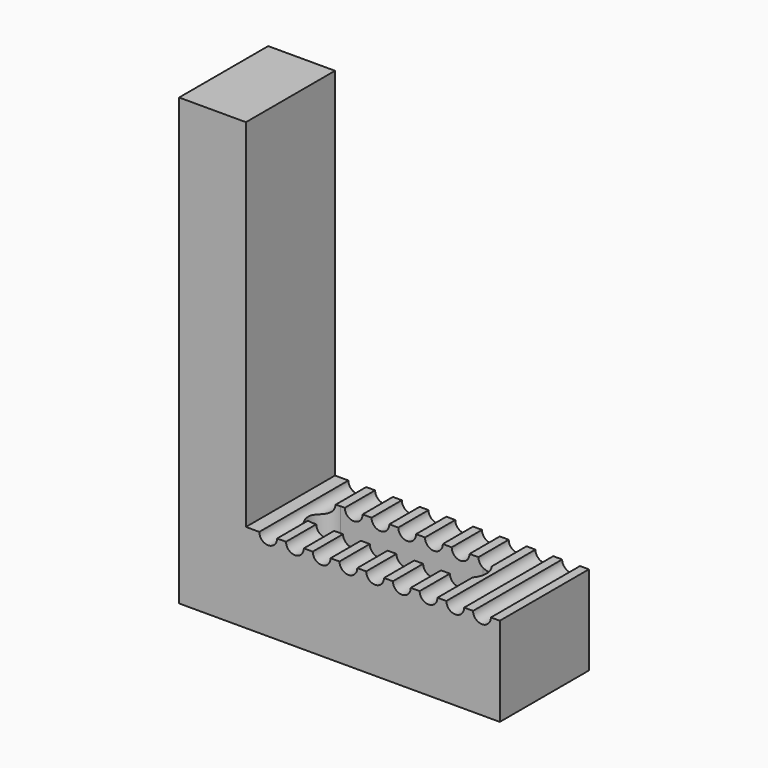
from build123d import *

# Parameters (mm, degrees)
F1_DEPTH = 15.875
F3_DEPTH = 25.4
F5_DEPTH = 25.4


with BuildPart() as f1:
    # F0 (on Front) → F1 (new body)
    with BuildSketch(Plane.XZ):
        Polygon((-45.72, 0), (0, 0), (0, 12.7), (-36.195, 12.7), (-36.195, 63.5), (-45.72, 63.5), align=None)
    extrude(amount=F1_DEPTH)

    # F2 (on face) → F3 (cut)
    with BuildSketch(Plane.XY.offset(12.7)):
        with BuildLine():
            Line((-10.795, -5.3975), (-31.115, -5.3975))
            ThreePointArc((-31.115, -5.3975), (-33.655, -7.9375), (-31.115, -10.4775))
            Line((-31.115, -10.4775), (-10.795, -10.4775))
            ThreePointArc((-10.795, -10.4775), (-8.255, -7.9375), (-10.795, -5.3975))
        make_face()
    extrude(amount=-F3_DEPTH, mode=Mode.SUBTRACT)

    # F4 (on face) → F5 (cut)
    with BuildSketch(Plane(origin=(0, 0, 0), x_dir=(-1, 0, 0), z_dir=(0, 1, 0))):
        with BuildLine():
            ThreePointArc((24.13, 12.7), (25.4, 11.43), (26.67, 12.7))
            Line((26.67, 12.7), (24.13, 12.7))
        make_face()
        with BuildLine():
            Line((30.48, 12.7), (27.94, 12.7))
            ThreePointArc((27.94, 12.7), (29.21, 11.43), (30.48, 12.7))
        make_face()
        with BuildLine():
            ThreePointArc((20.32, 12.7), (21.59, 11.43), (22.86, 12.7))
            Line((22.86, 12.7), (20.32, 12.7))
        make_face()
        with BuildLine():
            Line((34.29, 12.7), (31.75, 12.7))
            ThreePointArc((31.75, 12.7), (33.02, 11.43), (34.29, 12.7))
        make_face()
        with BuildLine():
            ThreePointArc((16.51, 12.7), (17.78, 11.43), (19.05, 12.7))
            Line((19.05, 12.7), (16.51, 12.7))
        make_face()
        with BuildLine():
            ThreePointArc((12.7, 12.7), (13.97, 11.43), (15.24, 12.7))
            Line((15.24, 12.7), (12.7, 12.7))
        make_face()
        with BuildLine():
            ThreePointArc((8.89, 12.7), (10.16, 11.43), (11.43, 12.7))
            Line((11.43, 12.7), (8.89, 12.7))
        make_face()
        with BuildLine():
            ThreePointArc((5.08, 12.7), (6.35, 11.43), (7.62, 12.7))
            Line((7.62, 12.7), (5.08, 12.7))
        make_face()
        with BuildLine():
            Line((3.81, 12.7), (1.27, 12.7))
            ThreePointArc((1.27, 12.7), (2.54, 11.43), (3.81, 12.7))
        make_face()
        with BuildLine():
            ThreePointArc((3.81, 12.7), (2.54, 13.97), (1.27, 12.7))
            Line((1.27, 12.7), (3.81, 12.7))
        make_face()
    extrude(amount=-F5_DEPTH, mode=Mode.SUBTRACT)


solid = f1.part
